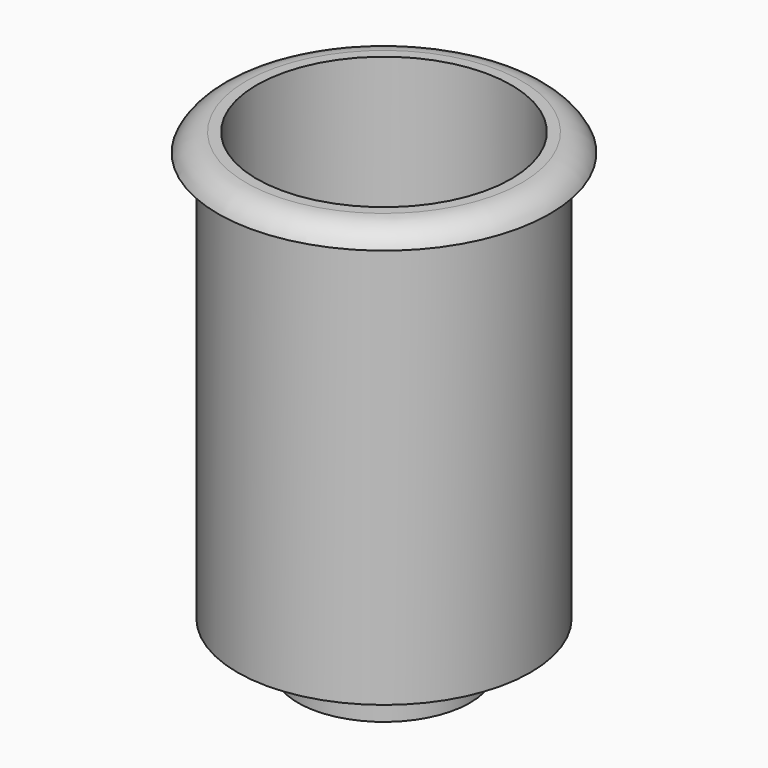
from build123d import *


# Not quite as in the source:
# - a fillet or chamfer that OpenCascade refuses, or shapes differently, is made with other operations: its cross-section is extruded or revolved along the edge and cut away or added


with BuildPart() as f1:
    # F0 (on Front) → F1 (revolve)
    with BuildSketch(Plane.XZ):
        Polygon((-3.0760182999, 0), (0, 0), (0, 7.6753781177), (10.0012486801, 7.6753781177), (10.0012486801, 75.3582566977), (13.1937107071, 75.3582566977), (13.1937107071, 78.3602893353), (6.8093864247, 78.3602893353), (6.8093864247, 10.8100166544), (-3.0760182999, 10.8100166544), align=None)
    revolve(axis=Axis((-14.1970999539, 0, 39.5920351148), (0, 0, 1)))

    # F2: fillet of radius 5.08 on 1 edges, made by hand

    # F2_s1 → F2_t2 (revolve, cut)
    with BuildSketch(Plane.XZ):
        with BuildLine():
            ThreePointArc((13.1937107071, 75.3582566977), (11.3195166688, 77.544235524), (8.5581469182, 78.3602893353))
            Line((8.5581469182, 78.3602893353), (13.1937107071, 78.3602893353))
            Line((13.1937107071, 78.3602893353), (13.1937107071, 75.3582566977))
        make_face()
    revolve(axis=Axis((-14.1970999539, 0, 78.3602893353), (0, 0, 1)), mode=Mode.SUBTRACT)


solid = f1.part
